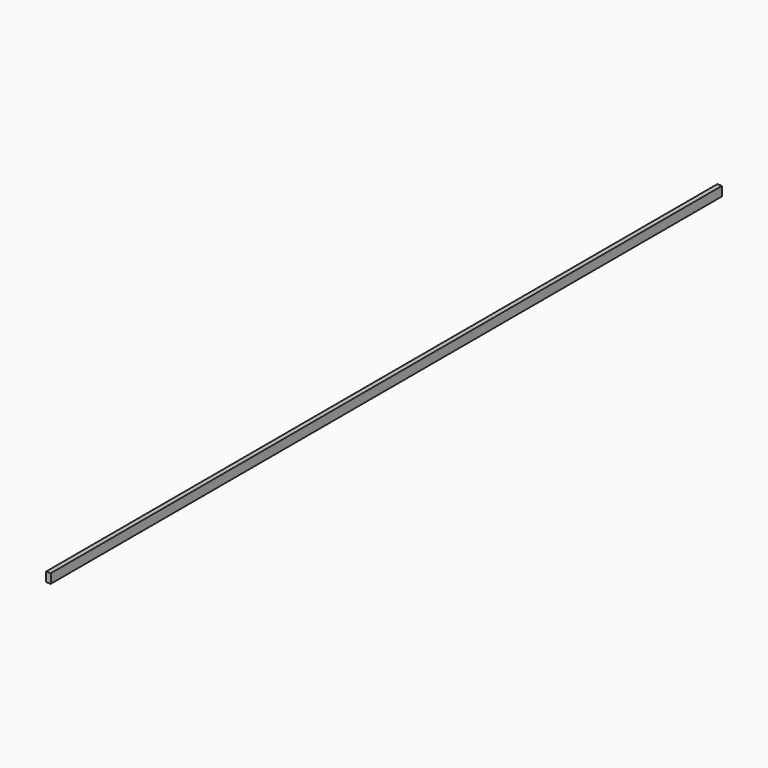
from build123d import *

# Parameters (mm, degrees)
F0_W     = 15.875
F0_H     = 31.75
F1_DEPTH = 2851.15


# Not quite as in the source:
# - a feature names something its author has since deleted; it is built from what else it names


with BuildPart() as f1:
    # F0 (on Front) → F1 (new body)
    with BuildSketch(Plane.XZ):
        with Locations((7.9375, -15.875)):
            Rectangle(F0_W, F0_H)
    extrude(amount=-F1_DEPTH)


solid = f1.part
